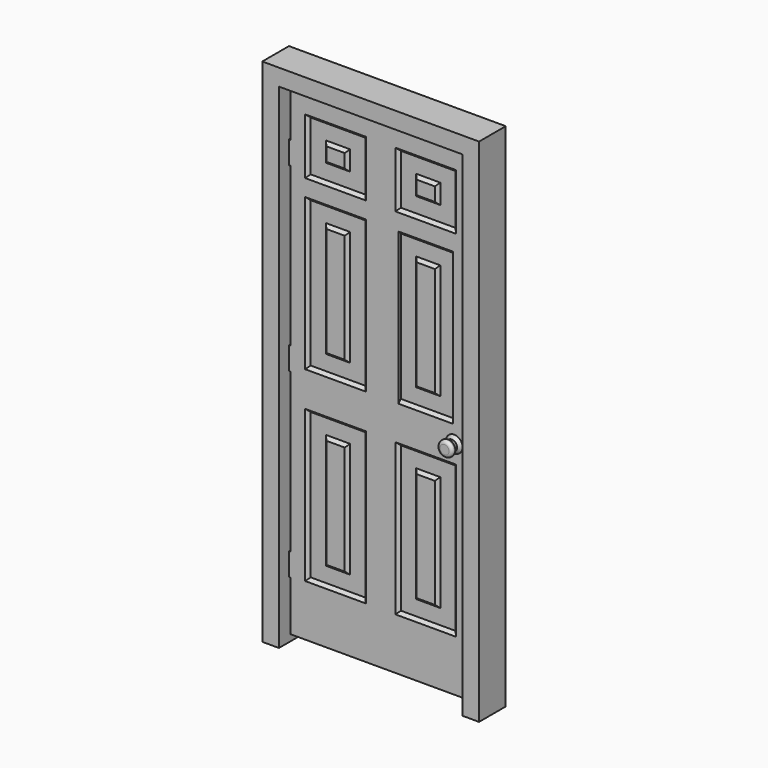
from build123d import *

# Parameters (mm, degrees)
F1_DEPTH  = 69.85
F2_DEPTH  = 17.4625
F3_W      = 228.6
F3_H      = 209.55
F3_W_2    = 101.6
F3_H_2    = 82.55
F3_H_3    = 609.6
F3_H_4    = 482.6
F4_DEPTH  = 12.7
F5_SIZE   = 12.69999
F6_W      = 228.6
F6_H      = 209.55
F6_W_2    = 101.6
F6_H_2    = 82.55
F6_H_3    = 609.6
F6_H_4    = 482.6
F7_DEPTH  = 12.7
F8_SIZE   = 12.69999
F9_R      = 34.925
F10_DEPTH = 12.7
F11_SIZE  = 12.69999
F12_R     = 9.525
F13_DEPTH = 12.7
F14_R     = 31.75
F14_R_2   = 9.525
F15_DEPTH = 25.4
F16_R     = 12.69999
F17_R     = 34.925
F18_DEPTH = 12.7
F19_SIZE  = 12.69999
F20_R     = 9.525
F21_DEPTH = 12.7
F22_R     = 31.75
F22_R_2   = 9.525
F23_DEPTH = 25.4
F24_R     = 12.69999


# Not quite as in the source:
# - a fillet or chamfer is up to 0.001 mm smaller than in the source, because OpenCascade refuses the exact size


with BuildPart() as f1:
    # F0 (on Front) → F1 (new body, symmetric)
    with BuildSketch(Plane.XZ):
        Polygon((454.025, 1069.975), (-454.025, 1069.975), (-454.025, -1069.975), (-384.175, -1069.975), (-384.175, -828.675), (-384.175, -733.425), (-384.175, -69.85), (-384.175, 25.4), (-384.175, 688.975), (-384.175, 784.225), (-384.175, 1000.125), (384.175, 1000.125), (384.175, -1069.975), (454.025, -1069.975), align=None)
    extrude(amount=F1_DEPTH, both=True)

    # F0 (on Front) → F2 (join, symmetric)
    with BuildSketch(Plane.XZ):
        Polygon((-384.175, -733.425), (-384.175, -828.675), (-377.825, -828.675), (-377.825, -1038.225), (377.825, -1038.225), (377.825, 993.775), (-377.825, 993.775), (-377.825, 784.225), (-384.175, 784.225), (-384.175, 688.975), (-377.825, 688.975), (-377.825, 25.4), (-384.175, 25.4), (-384.175, -69.85), (-377.825, -69.85), (-377.825, -733.425), align=None)
    extrude(amount=F2_DEPTH, both=True)

    # F3 (on face) → F4 (cut)
    with BuildSketch(Plane.XZ.offset(17.4625)):
        with Locations((-188.9125, 781.05)):
            Rectangle(F3_W, F3_H)
        with Locations((-188.9125, 781.05)):
            Rectangle(F3_W_2, F3_H_2, mode=Mode.SUBTRACT)
        with Locations((-188.9125, 276.225)):
            Rectangle(F3_W, F3_H_3)
        with Locations((-188.9125, 276.225)):
            Rectangle(F3_W_2, F3_H_4, mode=Mode.SUBTRACT)
        with Locations((188.9125, 781.05)):
            Rectangle(F3_W, F3_H)
        with Locations((188.9125, 781.05)):
            Rectangle(F3_W_2, F3_H_2, mode=Mode.SUBTRACT)
        with Locations((188.9125, 276.225)):
            Rectangle(F3_W, F3_H_3)
        with Locations((188.9125, 276.225)):
            Rectangle(F3_W_2, F3_H_4, mode=Mode.SUBTRACT)
        with Locations((-188.9125, -504.825)):
            Rectangle(F3_W, F3_H_3)
        with Locations((-188.9125, -504.825)):
            Rectangle(F3_W_2, F3_H_4, mode=Mode.SUBTRACT)
        with Locations((188.9125, -504.825)):
            Rectangle(F3_W, F3_H_3)
        with Locations((188.9125, -504.825)):
            Rectangle(F3_W_2, F3_H_4, mode=Mode.SUBTRACT)
    extrude(amount=-F4_DEPTH, mode=Mode.SUBTRACT)

    # F5 (size 12.7 in the source; OpenCascade refuses exactly that, so slightly less here)
    f5_edges = [f1.edges().sort_by_distance(p)[0] for p in [
        (-239.7125, -17.4625, 276.225),
        (-188.9125, -17.4625, 517.525),
        (-138.1125, -17.4625, 276.225),
        (-188.9125, -17.4625, 34.925),
        (-239.7125, -17.4625, 781.05),
        (-188.9125, -17.4625, 822.325),
        (-138.1125, -17.4625, 781.05),
        (-188.9125, -17.4625, 739.775),
        (188.9125, -17.4625, 822.325),
        (239.7125, -17.4625, 781.05),
        (188.9125, -17.4625, 739.775),
        (138.1125, -17.4625, 781.05),
        (138.1125, -17.4625, 276.225),
        (188.9125, -17.4625, 517.525),
        (239.7125, -17.4625, 276.225),
        (188.9125, -17.4625, 34.925),
        (-239.7125, -17.4625, -504.825),
        (-188.9125, -17.4625, -263.525),
        (-138.1125, -17.4625, -504.825),
        (-188.9125, -17.4625, -746.125),
        (188.9125, -17.4625, -263.525),
        (239.7125, -17.4625, -504.825),
        (188.9125, -17.4625, -746.125),
        (138.1125, -17.4625, -504.825),
        (-303.2125, -17.4625, 781.05),
        (-188.9125, -17.4625, 885.825),
        (-74.6125, -17.4625, 781.05),
        (-188.9125, -17.4625, 676.275),
        (-188.9125, -17.4625, 581.025),
        (-303.2125, -17.4625, 276.225),
        (-74.6125, -17.4625, 276.225),
        (74.6125, -17.4625, 781.05),
        (188.9125, -17.4625, 885.825),
        (303.2125, -17.4625, 781.05),
        (188.9125, -17.4625, 676.275),
        (188.9125, -17.4625, 581.025),
        (-188.9125, -17.4625, -28.575),
        (188.9125, -17.4625, -28.575),
        (-188.9125, -17.4625, -200.025),
        (-303.2125, -17.4625, -504.825),
        (-74.6125, -17.4625, -504.825),
        (188.9125, -17.4625, -200.025),
        (74.6125, -17.4625, -504.825),
        (303.2125, -17.4625, -504.825),
        (-188.9125, -17.4625, -809.625),
        (188.9125, -17.4625, -809.625),
    ]]
    chamfer(f5_edges, length=F5_SIZE)

    # F6 (on face) → F7 (cut)
    with BuildSketch(Plane(origin=(0, 17.4625, 0), x_dir=(-1, 0, 0), z_dir=(0, 1, 0))):
        with Locations((-188.462795082, 793.75)):
            Rectangle(F6_W, F6_H)
        with Locations((-188.462795082, 793.75)):
            Rectangle(F6_W_2, F6_H_2, mode=Mode.SUBTRACT)
        with Locations((189.362204918, 793.75)):
            Rectangle(F6_W, F6_H)
        with Locations((189.362204918, 793.75)):
            Rectangle(F6_W_2, F6_H_2, mode=Mode.SUBTRACT)
        with Locations((-188.462795082, 288.925)):
            Rectangle(F6_W, F6_H_3)
        with Locations((-188.462795082, 288.925)):
            Rectangle(F6_W_2, F6_H_4, mode=Mode.SUBTRACT)
        with Locations((189.362204918, 288.925)):
            Rectangle(F6_W, F6_H_3)
        with Locations((189.362204918, 288.925)):
            Rectangle(F6_W_2, F6_H_4, mode=Mode.SUBTRACT)
        with Locations((189.362204918, -492.125)):
            Rectangle(F6_W, F6_H_3)
        with Locations((189.362204918, -492.125)):
            Rectangle(F6_W_2, F6_H_4, mode=Mode.SUBTRACT)
        with Locations((-188.462795082, -492.125)):
            Rectangle(F6_W, F6_H_3)
        with Locations((-188.462795082, -492.125)):
            Rectangle(F6_W_2, F6_H_4, mode=Mode.SUBTRACT)
    extrude(amount=-F7_DEPTH, mode=Mode.SUBTRACT)

    # F8 (size 12.7 in the source; OpenCascade refuses exactly that, so slightly less here)
    f8_edges = [f1.edges().sort_by_distance(p)[0] for p in [
        (137.662795, 17.4625, 793.75),
        (188.462795, 17.4625, 835.025),
        (239.262795, 17.4625, 793.75),
        (188.462795, 17.4625, 752.475),
        (-240.162205, 17.4625, 793.75),
        (-189.362205, 17.4625, 835.025),
        (-138.562205, 17.4625, 793.75),
        (-189.362205, 17.4625, 752.475),
        (137.662795, 17.4625, 288.925),
        (188.462795, 17.4625, 530.225),
        (239.262795, 17.4625, 288.925),
        (188.462795, 17.4625, 47.625),
        (-240.162205, 17.4625, 288.925),
        (-189.362205, 17.4625, 530.225),
        (-138.562205, 17.4625, 288.925),
        (-189.362205, 17.4625, 47.625),
        (188.462795, 17.4625, -250.825),
        (239.262795, 17.4625, -492.125),
        (188.462795, 17.4625, -733.425),
        (137.662795, 17.4625, -492.125),
        (-240.162205, 17.4625, -492.125),
        (-189.362205, 17.4625, -250.825),
        (-138.562205, 17.4625, -492.125),
        (-189.362205, 17.4625, -733.425),
        (188.462795, 17.4625, 688.975),
        (302.762795, 17.4625, 793.75),
        (188.462795, 17.4625, 898.525),
        (74.162795, 17.4625, 793.75),
        (-75.062205, 17.4625, 793.75),
        (-189.362205, 17.4625, 898.525),
        (-303.662205, 17.4625, 793.75),
        (-189.362205, 17.4625, 688.975),
        (188.462795, 17.4625, 593.725),
        (302.762795, 17.4625, 288.925),
        (74.162795, 17.4625, 288.925),
        (-75.062205, 17.4625, 288.925),
        (-189.362205, 17.4625, 593.725),
        (-303.662205, 17.4625, 288.925),
        (-189.362205, 17.4625, -15.875),
        (188.462795, 17.4625, -15.875),
        (188.462795, 17.4625, -187.325),
        (302.762795, 17.4625, -492.125),
        (74.162795, 17.4625, -492.125),
        (-75.062205, 17.4625, -492.125),
        (-189.362205, 17.4625, -187.325),
        (-303.662205, 17.4625, -492.125),
        (-189.362205, 17.4625, -796.925),
        (188.462795, 17.4625, -796.925),
    ]]
    chamfer(f8_edges, length=F8_SIZE)

    # F9 (on face) → F10 (join)
    with BuildSketch(Plane.XZ.offset(17.4625)):
        with Locations((307.975, -114.3)):
            Circle(F9_R)
    extrude(amount=F10_DEPTH)

    # F11 (size 12.7 in the source; OpenCascade refuses exactly that, so slightly less here)
    f11_edges = [f1.edges().sort_by_distance(p)[0] for p in [
        (273.05, -30.1625, -114.3),
    ]]
    chamfer(f11_edges, length=F11_SIZE)

    # F12 (on face) → F13 (join)
    with BuildSketch(Plane.XZ.offset(30.1625)):
        with Locations((307.975, -114.3)):
            Circle(F12_R)
    extrude(amount=F13_DEPTH)

    # F14 (on face) → F15 (join)
    with BuildSketch(Plane.XZ.offset(42.8625)):
        with Locations((307.975, -114.3)):
            Circle(F14_R)
        with Locations((307.975, -114.3)):
            Circle(F14_R_2, mode=Mode.SUBTRACT)
        with Locations((307.975, -114.3)):
            Circle(F14_R_2)
    extrude(amount=F15_DEPTH)

    # F16 (radius 12.7 in the source; OpenCascade refuses exactly that, so slightly less here)
    f16_edges = [f1.edges().sort_by_distance(p)[0] for p in [
        (339.725, -55.5625, -114.3),
        (276.225, -42.8625, -114.3),
        (276.225, -68.2625, -114.3),
    ]]
    fillet(f16_edges, radius=F16_R)

    # F17 (on face) → F18 (join)
    with BuildSketch(Plane(origin=(0, 17.4625, 0), x_dir=(-1, 0, 0), z_dir=(0, 1, 0))):
        with Locations((-307.975, -101.6)):
            Circle(F17_R)
    extrude(amount=F18_DEPTH)

    # F19 (size 12.7 in the source; OpenCascade refuses exactly that, so slightly less here)
    f19_edges = [f1.edges().sort_by_distance(p)[0] for p in [
        (342.9, 30.1625, -101.6),
    ]]
    chamfer(f19_edges, length=F19_SIZE)

    # F20 (on face) → F21 (join)
    with BuildSketch(Plane(origin=(0, 30.1625, 0), x_dir=(-1, 0, 0), z_dir=(0, 1, 0))):
        with Locations((-307.975, -101.6)):
            Circle(F20_R)
    extrude(amount=F21_DEPTH)

    # F22 (on face) → F23 (join)
    with BuildSketch(Plane(origin=(0, 42.8625, 0), x_dir=(-1, 0, 0), z_dir=(0, 1, 0))):
        with Locations((-307.975, -101.6)):
            Circle(F22_R)
        with Locations((-307.975, -101.6)):
            Circle(F22_R_2, mode=Mode.SUBTRACT)
        with Locations((-307.975, -101.6)):
            Circle(F22_R_2)
    extrude(amount=F23_DEPTH)

    # F24 (radius 12.7 in the source; OpenCascade refuses exactly that, so slightly less here)
    f24_edges = [f1.edges().sort_by_distance(p)[0] for p in [
        (276.225, 55.5625, -101.6),
        (339.725, 42.8625, -101.6),
        (339.725, 68.2625, -101.6),
    ]]
    fillet(f24_edges, radius=F24_R)


solid = f1.part
